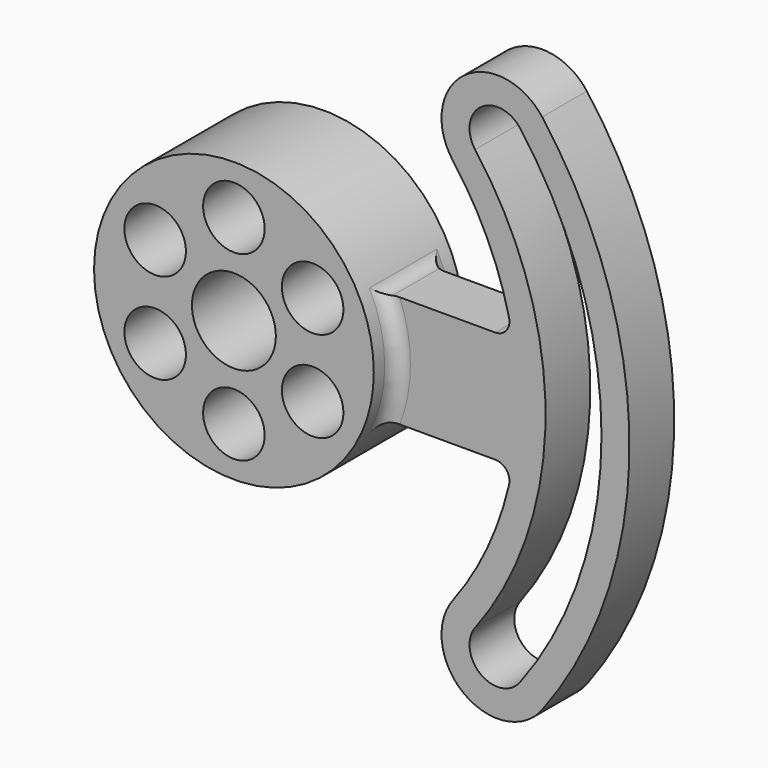
from build123d import *

# Parameters (mm, degrees)
F0_R         = 11
F0_R_2       = 15
F1_DEPTH     = 20
F2_DEPTH     = 10
F3_T1_DEPTH  = 10
F3_T3_DEPTH  = 10
F3_T5_DEPTH  = 20
F3_T10_ANGLE = 38.1317076079
F3_T15_ANGLE = 38.1317076079
F3_T20_ANGLE = 38.1317076079
F3_T25_ANGLE = 38.1317076079
F3_T31_DEPTH = 18.0325080763
F3_T35_ANGLE = 38.1317076079
F3_T42_DEPTH = 18.0325080763
F3_T46_ANGLE = 38.1317076079
F3_T53_DEPTH = 18.0325080763
F3_T57_ANGLE = 38.1317076079
F3_T64_DEPTH = 18.0325080763
F3_T68_ANGLE = 38.1317076079


# Not quite as in the source:
# - a fillet or chamfer that OpenCascade refuses, or shapes differently, is made with other operations: its cross-section is extruded or revolved along the edge and cut away or added


with BuildPart() as f1:
    # F0 (on Front) → F1 (new body, symmetric)
    with BuildSketch(Plane.XZ):
        with BuildLine():
            ThreePointArc((45.8257569496, -20), (48.9453156465, -10.2154821845), (50, 0))
            ThreePointArc((50, 0), (48.9453156465, 10.2154821845), (45.8257569496, 20))
            ThreePointArc((45.8257569496, 20), (-50, 0), (45.8257569496, -20))
        make_face()
        with Locations((-28.145825623, -16.25)):
            Circle(F0_R, mode=Mode.SUBTRACT)
        with Locations((0, -32.5)):
            Circle(F0_R, mode=Mode.SUBTRACT)
        with Locations((28.145825623, -16.25)):
            Circle(F0_R, mode=Mode.SUBTRACT)
        with Locations((-28.145825623, 16.25)):
            Circle(F0_R, mode=Mode.SUBTRACT)
        Circle(F0_R_2, mode=Mode.SUBTRACT)
        with Locations((28.145825623, 16.25)):
            Circle(F0_R, mode=Mode.SUBTRACT)
        with Locations((0, 32.5)):
            Circle(F0_R, mode=Mode.SUBTRACT)
    extrude(amount=F1_DEPTH, both=True)

    # F0 (on Front) → F2 (join, symmetric)
    with BuildSketch(Plane.XZ):
        with BuildLine():
            ThreePointArc((45.8257569496, -20), (48.9453156465, -10.2154821845), (50, 0))
            ThreePointArc((50, 0), (48.9453156465, 10.2154821845), (45.8257569496, 20))
            ThreePointArc((45.8257569496, 20), (-50, 0), (45.8257569496, -20))
        make_face()
        with Locations((-28.145825623, -16.25)):
            Circle(F0_R, mode=Mode.SUBTRACT)
        with Locations((0, -32.5)):
            Circle(F0_R, mode=Mode.SUBTRACT)
        with Locations((28.145825623, -16.25)):
            Circle(F0_R, mode=Mode.SUBTRACT)
        with Locations((-28.145825623, 16.25)):
            Circle(F0_R, mode=Mode.SUBTRACT)
        Circle(F0_R_2, mode=Mode.SUBTRACT)
        with Locations((28.145825623, 16.25)):
            Circle(F0_R, mode=Mode.SUBTRACT)
        with Locations((0, 32.5)):
            Circle(F0_R, mode=Mode.SUBTRACT)
        with BuildLine():
            ThreePointArc((45.8257569496, 20), (48.9453156465, 10.2154821845), (50, 0))
            ThreePointArc((50, 0), (48.9453156465, -10.2154821845), (45.8257569496, -20))
            Line((45.8257569496, -20), (91.6475165291, -20))
            ThreePointArc((91.6475165291, -20), (83.8557409084, -45.8703249329), (70.2430836554, -69.2087276625))
            ThreePointArc((70.2430836554, -69.2087276625), (74.1794933933, -97.2177383265), (102.1885040573, -93.2813285886))
            ThreePointArc((102.1885040573, -93.2813285886), (133.4, 0), (102.1885040573, 93.2813285886))
            ThreePointArc((102.1885040573, 93.2813285886), (74.1794933933, 97.2177383265), (70.2430836554, 69.2087276625))
            ThreePointArc((70.2430836554, 69.2087276625), (83.8557409084, 45.8703249329), (91.6475165291, 20))
            Line((91.6475165291, 20), (45.8257569496, 20))
        make_face()
        with BuildLine():
            ThreePointArc((94.2021489569, -87.263178357), (80.1976436249, -89.231383226), (78.2294387559, -75.226877894))
            ThreePointArc((78.2294387559, -75.226877894), (103.4, 0), (78.2294387559, 75.226877894))
            ThreePointArc((78.2294387559, 75.226877894), (80.1976436249, 89.231383226), (94.2021489569, 87.263178357))
            ThreePointArc((94.2021489569, 87.263178357), (123.4, 0), (94.2021489569, -87.263178357))
        make_face(mode=Mode.SUBTRACT)
    extrude(amount=F2_DEPTH, both=True)

    # F3: fillet of radius 5.08 on 10 edges, made by hand

    # F3_s2 → F3_t1 (join)
    with BuildSketch(Plane.XZ.offset(-10)):
        with BuildLine():
            ThreePointArc((44.5159406137, 22.7668845316), (46.3877440145, 20.7465818007), (49.0387601801, 20))
            Line((49.0387601801, 20), (45.8257569496, 20))
            ThreePointArc((45.8257569496, 20), (45.1920290777, 21.3934688128), (44.5159406137, 22.7668845316))
        make_face()
        with BuildLine():
            ThreePointArc((44.5159406137, -22.7668845316), (46.3877440145, -20.7465818007), (49.0387601801, -20))
            Line((49.0387601801, -20), (45.8257569496, -20))
            ThreePointArc((45.8257569496, -20), (45.1920290777, -21.3934688128), (44.5159406137, -22.7668845316))
        make_face()
    extrude(amount=F3_T1_DEPTH)

    # F3_s4 → F3_t3 (join)
    with BuildSketch(Plane.XZ):
        with BuildLine():
            ThreePointArc((44.5159406137, 22.7668845316), (46.3877440145, 20.7465818007), (49.0387601801, 20))
            Line((49.0387601801, 20), (45.8257569496, 20))
            ThreePointArc((45.8257569496, 20), (45.1920290777, 21.3934688128), (44.5159406137, 22.7668845316))
        make_face()
        with BuildLine():
            ThreePointArc((44.5159406137, -22.7668845316), (46.3877440145, -20.7465818007), (49.0387601801, -20))
            Line((49.0387601801, -20), (45.8257569496, -20))
            ThreePointArc((45.8257569496, -20), (45.1920290777, -21.3934688128), (44.5159406137, -22.7668845316))
        make_face()
    extrude(amount=F3_T3_DEPTH)

    # F3_s6 → F3_t5 (join)
    with BuildSketch(Plane.XZ.offset(-10)):
        with BuildLine():
            ThreePointArc((85.4205587726, -20), (89.4014218376, -21.924191188), (90.3665598512, -26.2390829694))
            ThreePointArc((90.3665598512, -26.2390829694), (91.0502400753, -23.1284113368), (91.6475165291, -20))
            Line((91.6475165291, -20), (85.4205587726, -20))
        make_face()
        with BuildLine():
            ThreePointArc((85.4205587726, 20), (89.4014218376, 21.924191188), (90.3665598512, 26.2390829694))
            ThreePointArc((90.3665598512, 26.2390829694), (91.0502400753, 23.1284113368), (91.6475165291, 20))
            Line((91.6475165291, 20), (85.4205587726, 20))
        make_face()
    extrude(amount=F3_T5_DEPTH)


with BuildPart() as f3_tool8:
    # F3_s9 → F3_t10 (revolve)
    with BuildSketch(Plane(origin=(0, 0, 0), x_dir=(0, 1, 0), z_dir=(-0.6174712722, 0, -0.7865934325))):
        with BuildLine():
            ThreePointArc((10, 55.08), (11.4878975516, 51.4878975516), (15.08, 50))
            Line((15.08, 50), (10, 50))
            Line((10, 50), (10, 55.08))
        make_face()
    revolve(axis=Axis((0, 10, 0), (0, -1, 0)), revolution_arc=F3_T10_ANGLE)

    split(bisect_by=Plane.XY.offset(-20), keep=Keep.TOP)


with BuildPart() as f1_1:
    add(f1.part)

    # F3_t7: union F3_tool8
    add(f3_tool8.part)


with BuildPart() as f3_tool13:
    # F3_s14 → F3_t15 (revolve)
    with BuildSketch(Plane.XY):
        with BuildLine():
            ThreePointArc((55.08, 10), (51.4878975516, 11.4878975516), (50, 15.08))
            Line((50, 15.08), (50, 10))
            Line((50, 10), (55.08, 10))
        make_face()
    revolve(axis=Axis((0, 10, 0), (0, -1, 0)), revolution_arc=F3_T15_ANGLE)

    split(bisect_by=Plane.XY.offset(20), keep=Keep.BOTTOM)


with BuildPart() as f1_2:
    add(f1_1.part)

    # F3_t12: union F3_tool13
    add(f3_tool13.part)


with BuildPart() as f3_tool18:
    # F3_s19 → F3_t20 (revolve)
    with BuildSketch(Plane.XY):
        with BuildLine():
            ThreePointArc((55.08, -10), (51.4878975516, -11.4878975516), (50, -15.08))
            Line((50, -15.08), (50, -10))
            Line((50, -10), (55.08, -10))
        make_face()
    revolve(axis=Axis((0, -10, 0), (0, 1, 0)), revolution_arc=F3_T20_ANGLE)

    split(bisect_by=Plane.XY.offset(-20), keep=Keep.TOP)


with BuildPart() as f1_3:
    add(f1_2.part)

    # F3_t17: union F3_tool18
    add(f3_tool18.part)


with BuildPart() as f3_tool23:
    # F3_s24 → F3_t25 (revolve)
    with BuildSketch(Plane(origin=(0, 0, 0), x_dir=(0, 1, 0), z_dir=(-0.6174712722, 0, 0.7865934325))):
        with BuildLine():
            ThreePointArc((-10, -55.08), (-11.4878975516, -51.4878975516), (-15.08, -50))
            Line((-15.08, -50), (-10, -50))
            Line((-10, -50), (-10, -55.08))
        make_face()
    revolve(axis=Axis((0, -10, 0), (0, 1, 0)), revolution_arc=F3_T25_ANGLE)

    split(bisect_by=Plane.XY.offset(20), keep=Keep.BOTTOM)


with BuildPart() as f1_4:
    add(f1_3.part)

    # F3_t22: union F3_tool23
    add(f3_tool23.part)


with BuildPart() as f3_tool29:
    # F3_s30 → F3_t31 (new body)
    with BuildSketch(Plane.XZ):
        with BuildLine():
            ThreePointArc((44.5159406137, 22.7668845316), (46.3877440145, 20.7465818007), (49.0387601801, 20))
            Line((49.0387601801, 20), (45.8257569496, 20))
            ThreePointArc((45.8257569496, 20), (45.1920290777, 21.3934688128), (44.5159406137, 22.7668845316))
        make_face()
    extrude(amount=-F3_T31_DEPTH)

    split(bisect_by=Plane.XZ.offset(-10), keep=Keep.BOTTOM)


with BuildPart() as f3_tool33:
    # F3_s34 → F3_t35 (revolve)
    with BuildSketch(Plane.XY):
        with BuildLine():
            ThreePointArc((55.08, 10), (51.4878975516, 11.4878975516), (50, 15.08))
            Line((50, 15.08), (50, 10))
            Line((50, 10), (55.08, 10))
        make_face()
    revolve(axis=Axis((0, 10, 0), (0, -1, 0)), revolution_arc=F3_T35_ANGLE)

    split(bisect_by=Plane.XY.offset(20), keep=Keep.TOP)


with BuildPart() as f3_tool29_1:
    add(f3_tool29.part)

    # F3_t37: intersect F3_tool33
    add(f3_tool33.part, mode=Mode.INTERSECT)


with BuildPart() as f1_5:
    add(f1_4.part)

    # F3_t27: union F3_tool29
    add(f3_tool29_1.part)


with BuildPart() as f3_tool40:
    # F3_s41 → F3_t42 (new body)
    with BuildSketch(Plane.XZ):
        with BuildLine():
            ThreePointArc((44.5159406137, 22.7668845316), (46.3877440145, 20.7465818007), (49.0387601801, 20))
            Line((49.0387601801, 20), (45.8257569496, 20))
            ThreePointArc((45.8257569496, 20), (45.1920290777, 21.3934688128), (44.5159406137, 22.7668845316))
        make_face()
    extrude(amount=F3_T42_DEPTH)

    split(bisect_by=Plane.XZ.offset(10), keep=Keep.TOP)


with BuildPart() as f3_tool44:
    # F3_s45 → F3_t46 (revolve)
    with BuildSketch(Plane(origin=(0, 0, 0), x_dir=(0, 1, 0), z_dir=(-0.6174712722, 0, 0.7865934325))):
        with BuildLine():
            ThreePointArc((-10, -55.08), (-11.4878975516, -51.4878975516), (-15.08, -50))
            Line((-15.08, -50), (-10, -50))
            Line((-10, -50), (-10, -55.08))
        make_face()
    revolve(axis=Axis((0, -10, 0), (0, 1, 0)), revolution_arc=F3_T46_ANGLE)

    split(bisect_by=Plane.XY.offset(20), keep=Keep.TOP)


with BuildPart() as f3_tool40_1:
    add(f3_tool40.part)

    # F3_t48: intersect F3_tool44
    add(f3_tool44.part, mode=Mode.INTERSECT)


with BuildPart() as f1_6:
    add(f1_5.part)

    # F3_t38: union F3_tool40
    add(f3_tool40_1.part)


with BuildPart() as f3_tool51:
    # F3_s52 → F3_t53 (new body)
    with BuildSketch(Plane.XZ):
        with BuildLine():
            ThreePointArc((44.5159406137, -22.7668845316), (46.3877440145, -20.7465818007), (49.0387601801, -20))
            Line((49.0387601801, -20), (45.8257569496, -20))
            ThreePointArc((45.8257569496, -20), (45.1920290777, -21.3934688128), (44.5159406137, -22.7668845316))
        make_face()
    extrude(amount=-F3_T53_DEPTH)

    split(bisect_by=Plane.XZ.offset(-10), keep=Keep.BOTTOM)


with BuildPart() as f3_tool55:
    # F3_s56 → F3_t57 (revolve)
    with BuildSketch(Plane(origin=(0, 0, 0), x_dir=(0, 1, 0), z_dir=(-0.6174712722, 0, -0.7865934325))):
        with BuildLine():
            ThreePointArc((10, 55.08), (11.4878975516, 51.4878975516), (15.08, 50))
            Line((15.08, 50), (10, 50))
            Line((10, 50), (10, 55.08))
        make_face()
    revolve(axis=Axis((0, 10, 0), (0, -1, 0)), revolution_arc=F3_T57_ANGLE)

    split(bisect_by=Plane.XY.offset(-20), keep=Keep.BOTTOM)


with BuildPart() as f3_tool51_1:
    add(f3_tool51.part)

    # F3_t59: intersect F3_tool55
    add(f3_tool55.part, mode=Mode.INTERSECT)


with BuildPart() as f1_7:
    add(f1_6.part)

    # F3_t49: union F3_tool51
    add(f3_tool51_1.part)


with BuildPart() as f3_tool62:
    # F3_s63 → F3_t64 (new body)
    with BuildSketch(Plane.XZ):
        with BuildLine():
            ThreePointArc((44.5159406137, -22.7668845316), (46.3877440145, -20.7465818007), (49.0387601801, -20))
            Line((49.0387601801, -20), (45.8257569496, -20))
            ThreePointArc((45.8257569496, -20), (45.1920290777, -21.3934688128), (44.5159406137, -22.7668845316))
        make_face()
    extrude(amount=F3_T64_DEPTH)

    split(bisect_by=Plane.XZ.offset(10), keep=Keep.TOP)


with BuildPart() as f3_tool66:
    # F3_s67 → F3_t68 (revolve)
    with BuildSketch(Plane.XY):
        with BuildLine():
            ThreePointArc((55.08, -10), (51.4878975516, -11.4878975516), (50, -15.08))
            Line((50, -15.08), (50, -10))
            Line((50, -10), (55.08, -10))
        make_face()
    revolve(axis=Axis((0, -10, 0), (0, 1, 0)), revolution_arc=F3_T68_ANGLE)

    split(bisect_by=Plane.XY.offset(-20), keep=Keep.BOTTOM)


with BuildPart() as f3_tool62_1:
    add(f3_tool62.part)

    # F3_t70: intersect F3_tool66
    add(f3_tool66.part, mode=Mode.INTERSECT)


with BuildPart() as f1_8:
    add(f1_7.part)

    # F3_t60: union F3_tool62
    add(f3_tool62_1.part)


solid = f1_8.part
